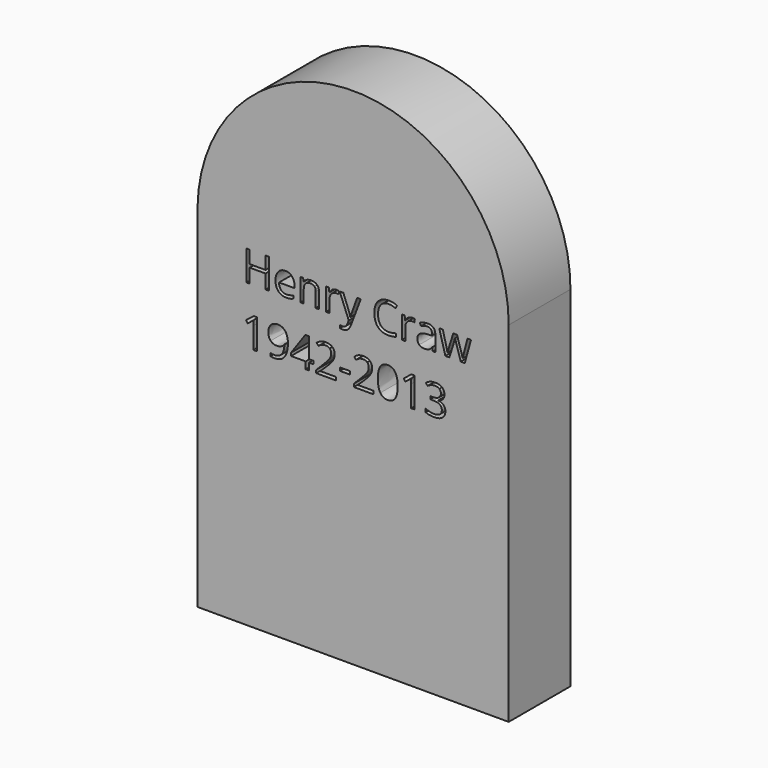
from build123d import *

# Parameters (mm, degrees)
F0_W     = 3.3136069849
F0_H     = 1.0260517065
F1_DEPTH = 25.4


with BuildPart() as f1:
    # F0 (on Front) → F1 (new body)
    with BuildSketch(Plane.XZ):
        with BuildLine():
            ThreePointArc((68.7805563211, 9.0927695855), (17.9996618483, 60.291606621), (-33.6136780679, 9.9320663139))
            Line((-33.6136780679, 9.9320663139), (-33.6136780679, -105.8909147978))
            Line((-33.6136780679, -105.8909147978), (68.7805563211, -105.8909147978))
            Line((68.7805563211, -105.8909147978), (68.7805563211, 9.0927695855))
        make_face()
        with BuildLine():
            Line((-14.1120249478, -15.5934271273), (-14.1120249478, -25.4629644899))
            Line((-14.1120249478, -25.4629644899), (-15.2050400289, -25.4629644899))
            Line((-15.2050400289, -25.4629644899), (-15.2050400289, -18.4296500551))
            add(Edge.make_bspline(
                [(-15.2050400289, -18.4296500551), (-15.2050400289, -17.5504857508), (-15.1510373075, -16.7685263449)],
                knots=[0, 0, 0, 1, 1, 1], degree=2))
            add(Edge.make_bspline(
                [(-15.1510373075, -16.7685263449), (-15.2914443831, -16.9110935294), (-15.4674932549, -17.0655413126)],
                knots=[0, 0, 0, 1, 1, 1], degree=2))
            add(Edge.make_bspline(
                [(-15.4674932549, -17.0655413126), (-15.6435421266, -17.2199890958), (-17.0735341892, -18.3821276603)],
                knots=[0, 0, 0, 1, 1, 1], degree=2))
            Line((-17.0735341892, -18.3821276603), (-17.6675641246, -17.6131289076))
            Line((-17.6675641246, -17.6131289076), (-15.0559925178, -15.5934271273))
            Line((-15.0559925178, -15.5934271273), (-14.1120249478, -15.5934271273))
        make_face(mode=Mode.SUBTRACT)
        Polygon((-10.0877421493, 3.2081603542), (-10.0877421493, -6.6613770083), (-11.2347599518, -6.6613770083), (-11.2347599518, -2.0171429681), (-16.4341419679, -2.0171429681), (-16.4341419679, -6.6613770083), (-17.5811597703, -6.6613770083), (-17.5811597703, 3.2081603542), (-16.4341419679, 3.2081603542), (-16.4341419679, -0.9910912616), (-11.2347599518, -0.9910912616), (-11.2347599518, 3.2081603542), align=None, mode=Mode.SUBTRACT)
        with BuildLine():
            add(Edge.make_bspline(
                [(-4.2759692725, -17.4738018864), (-3.8709488621, -18.462051688), (-3.8709488621, -19.8056393963)],
                knots=[0, 0, 0, 1, 1, 1], degree=2))
            add(Edge.make_bspline(
                [(-3.8709488621, -19.8056393963), (-3.8709488621, -25.5990513478), (-8.353174738, -25.5990513478)],
                knots=[0, 0, 0, 1, 1, 1], degree=2))
            add(Edge.make_bspline(
                [(-8.353174738, -25.5990513478), (-9.1372942527, -25.5990513478), (-9.5952373301, -25.4629644899)],
                knots=[0, 0, 0, 1, 1, 1], degree=2))
            Line((-9.5952373301, -25.4629644899), (-9.5952373301, -24.4973958313))
            add(Edge.make_bspline(
                [(-9.5952373301, -24.4973958313), (-9.0552101162, -24.6723646486), (-8.3682955, -24.6723646486)],
                knots=[0, 0, 0, 1, 1, 1], degree=2))
            add(Edge.make_bspline(
                [(-8.3682955, -24.6723646486), (-6.7482138581, -24.6723646486), (-5.9208921663, -23.6700741395)],
                knots=[0, 0, 0, 1, 1, 1], degree=2))
            add(Edge.make_bspline(
                [(-5.9208921663, -23.6700741395), (-5.0935704745, -22.6677836303), (-5.0201267734, -20.5962392376)],
                knots=[0, 0, 0, 1, 1, 1], degree=2))
            Line((-5.0201267734, -20.5962392376), (-5.1000508011, -20.5962392376))
            add(Edge.make_bspline(
                [(-5.1000508011, -20.5962392376), (-5.4715895243, -21.1557074312), (-6.0861404938, -21.4494822356)],
                knots=[0, 0, 0, 1, 1, 1], degree=2))
            add(Edge.make_bspline(
                [(-6.0861404938, -21.4494822356), (-6.7006914633, -21.74325704), (-7.469690216, -21.74325704)],
                knots=[0, 0, 0, 1, 1, 1], degree=2))
            add(Edge.make_bspline(
                [(-7.469690216, -21.74325704), (-8.7787161826, -21.74325704), (-9.5487949897, -20.9602175798)],
                knots=[0, 0, 0, 1, 1, 1], degree=2))
            add(Edge.make_bspline(
                [(-9.5487949897, -20.9602175798), (-10.3188737969, -20.1771781195), (-10.3188737969, -18.7731073632)],
                knots=[0, 0, 0, 1, 1, 1], degree=2))
            add(Edge.make_bspline(
                [(-10.3188737969, -18.7731073632), (-10.3188737969, -17.2351098578), (-9.4580704178, -16.3440649548)],
                knots=[0, 0, 0, 1, 1, 1], degree=2))
            add(Edge.make_bspline(
                [(-9.4580704178, -16.3440649548), (-8.5972670387, -15.4530200517), (-7.1931962824, -15.4530200517)],
                knots=[0, 0, 0, 1, 1, 1], degree=2))
            add(Edge.make_bspline(
                [(-7.1931962824, -15.4530200517), (-6.1865855556, -15.4530200517), (-5.4337876193, -15.9692860683)],
                knots=[0, 0, 0, 1, 1, 1], degree=2))
            add(Edge.make_bspline(
                [(-5.4337876193, -15.9692860683), (-4.680989683, -16.4855520848), (-4.2759692725, -17.4738018864)],
                knots=[0, 0, 0, 1, 1, 1], degree=2))
        make_face(mode=Mode.SUBTRACT)
        Polygon((4.4973128456, -22.1752788112), (4.4973128456, -23.1948501912), (3.0327590413, -23.1948501912), (3.0327590413, -25.4629644899), (1.95918494, -25.4629644899), (1.95918494, -23.1948501912), (-2.8405769378, -23.1948501912), (-2.8405769378, -22.2163208795), (1.8446991706, -15.5394244059), (3.0327590413, -15.5394244059), (3.0327590413, -22.1752788112), align=None, mode=Mode.SUBTRACT)
        with BuildLine():
            add(Edge.make_bspline(
                [(-3.1451522865, -6.6851382057), (-3.6743789562, -6.7974638662), (-4.4239367292, -6.7974638662)],
                knots=[0, 0, 0, 1, 1, 1], degree=2))
            add(Edge.make_bspline(
                [(-4.4239367292, -6.7974638662), (-6.0634593508, -6.7974638662), (-7.0128271929, -5.7973334659)],
                knots=[0, 0, 0, 1, 1, 1], degree=2))
            add(Edge.make_bspline(
                [(-7.0128271929, -5.7973334659), (-7.9621950351, -4.7972030657), (-7.9621950351, -3.023753695)],
                knots=[0, 0, 0, 1, 1, 1], degree=2))
            add(Edge.make_bspline(
                [(-7.9621950351, -3.023753695), (-7.9621950351, -1.2330234535), (-7.0808706219, -0.1799703862)],
                knots=[0, 0, 0, 1, 1, 1], degree=2))
            add(Edge.make_bspline(
                [(-7.0808706219, -0.1799703862), (-6.1995462087, 0.873082681), (-4.7133913159, 0.873082681)],
                knots=[0, 0, 0, 1, 1, 1], degree=2))
            add(Edge.make_bspline(
                [(-4.7133913159, 0.873082681), (-3.3244413215, 0.873082681), (-2.5144005006, -0.0417234194)],
                knots=[0, 0, 0, 1, 1, 1], degree=2))
            add(Edge.make_bspline(
                [(-2.5144005006, -0.0417234194), (-1.7043596796, -0.9565295199), (-1.7043596796, -2.4556450659)],
                knots=[0, 0, 0, 1, 1, 1], degree=2))
            Line((-1.7043596796, -2.4556450659), (-1.7043596796, -3.1641607706))
            Line((-1.7043596796, -3.1641607706), (-6.8000564706, -3.1641607706))
            add(Edge.make_bspline(
                [(-6.8000564706, -3.1641607706), (-6.7654947289, -4.4667064107), (-6.1412232696, -5.1417404282)],
                knots=[0, 0, 0, 1, 1, 1], degree=2))
            add(Edge.make_bspline(
                [(-6.1412232696, -5.1417404282), (-5.5169518102, -5.8167744456), (-4.3828946609, -5.8167744456)],
                knots=[0, 0, 0, 1, 1, 1], degree=2))
            add(Edge.make_bspline(
                [(-4.3828946609, -5.8167744456), (-3.1883544636, -5.8167744456), (-2.0218956814, -5.3177892999)],
                knots=[0, 0, 0, 1, 1, 1], degree=2))
            Line((-2.0218956814, -5.3177892999), (-2.0218956814, -6.3179197002))
            add(Edge.make_bspline(
                [(-2.0218956814, -6.3179197002), (-2.6159256168, -6.5728125452), (-3.1451522865, -6.6851382057)],
                knots=[0, 0, 0, 1, 1, 1], degree=2))
        make_face(mode=Mode.SUBTRACT)
        with BuildLine():
            Line((6.3917283122, -6.6613770083), (5.270631816, -6.6613770083))
            Line((5.270631816, -6.6613770083), (5.270631816, -1.8745757837))
            add(Edge.make_bspline(
                [(5.270631816, -1.8745757837), (5.270631816, -0.9716502819), (4.859131079, -0.5255878032)],
                knots=[0, 0, 0, 1, 1, 1], degree=2))
            add(Edge.make_bspline(
                [(4.859131079, -0.5255878032), (4.4476303419, -0.0795253244), (3.5684660376, -0.0795253244)],
                knots=[0, 0, 0, 1, 1, 1], degree=2))
            add(Edge.make_bspline(
                [(3.5684660376, -0.0795253244), (2.408487582, -0.0795253244), (1.868460368, -0.707036947)],
                knots=[0, 0, 0, 1, 1, 1], degree=2))
            add(Edge.make_bspline(
                [(1.868460368, -0.707036947), (1.328433154, -1.3345485697), (1.328433154, -2.7796613943)],
                knots=[0, 0, 0, 1, 1, 1], degree=2))
            Line((1.328433154, -2.7796613943), (1.328433154, -6.6613770083))
            Line((1.328433154, -6.6613770083), (0.2073366578, -6.6613770083))
            Line((0.2073366578, -6.6613770083), (0.2073366578, 0.7369958231))
            Line((0.2073366578, 0.7369958231), (1.118902595, 0.7369958231))
            Line((1.118902595, 0.7369958231), (1.3003517389, -0.2760952303))
            Line((1.3003517389, -0.2760952303), (1.3543544603, -0.2760952303))
            add(Edge.make_bspline(
                [(1.3543544603, -0.2760952303), (1.6999718772, 0.2704123102), (2.3210031733, 0.5717474956)],
                knots=[0, 0, 0, 1, 1, 1], degree=2))
            add(Edge.make_bspline(
                [(2.3210031733, 0.5717474956), (2.9420344694, 0.873082681), (3.7045528955, 0.873082681)],
                knots=[0, 0, 0, 1, 1, 1], degree=2))
            add(Edge.make_bspline(
                [(3.7045528955, 0.873082681), (5.0416602773, 0.873082681), (5.7166942948, 0.2282901875)],
                knots=[0, 0, 0, 1, 1, 1], degree=2))
            add(Edge.make_bspline(
                [(5.7166942948, 0.2282901875), (6.3917283122, -0.4165023059), (6.3917283122, -1.8356938242)],
                knots=[0, 0, 0, 1, 1, 1], degree=2))
            Line((6.3917283122, -1.8356938242), (6.3917283122, -6.6613770083))
        make_face(mode=Mode.SUBTRACT)
        with BuildLine():
            Line((11.9367277453, -24.4239521302), (11.9367277453, -25.4629644899))
            Line((11.9367277453, -25.4629644899), (5.4499208511, -25.4629644899))
            Line((5.4499208511, -25.4629644899), (5.4499208511, -24.4973958313))
            Line((5.4499208511, -24.4973958313), (8.0485318047, -21.8858242245))
            add(Edge.make_bspline(
                [(8.0485318047, -21.8858242245), (9.2365916754, -20.6826435918), (9.6146107252, -20.1696177385)],
                knots=[0, 0, 0, 1, 1, 1], degree=2))
            add(Edge.make_bspline(
                [(9.6146107252, -20.1696177385), (9.992629775, -19.6565918853), (10.1816392999, -19.1705673927)],
                knots=[0, 0, 0, 1, 1, 1], degree=2))
            add(Edge.make_bspline(
                [(10.1816392999, -19.1705673927), (10.3706488247, -18.6845429001), (10.3706488247, -18.1250747064)],
                knots=[0, 0, 0, 1, 1, 1], degree=2))
            add(Edge.make_bspline(
                [(10.3706488247, -18.1250747064), (10.3706488247, -17.3344748652), (9.8911046587, -16.87221157)],
                knots=[0, 0, 0, 1, 1, 1], degree=2))
            add(Edge.make_bspline(
                [(9.8911046587, -16.87221157), (9.4115604927, -16.4099482749), (8.5604776035, -16.4099482749)],
                knots=[0, 0, 0, 1, 1, 1], degree=2))
            add(Edge.make_bspline(
                [(8.5604776035, -16.4099482749), (7.9470066885, -16.4099482749), (7.3961789302, -16.6129985073)],
                knots=[0, 0, 0, 1, 1, 1], degree=2))
            add(Edge.make_bspline(
                [(7.3961789302, -16.6129985073), (6.845351172, -16.8160487398), (6.1713972089, -17.3495956272)],
                knots=[0, 0, 0, 1, 1, 1], degree=2))
            Line((6.1713972089, -17.3495956272), (5.5773672736, -16.587077201))
            add(Edge.make_bspline(
                [(5.5773672736, -16.587077201), (6.9403959616, -15.4530200517), (8.5475169504, -15.4530200517)],
                knots=[0, 0, 0, 1, 1, 1], degree=2))
            add(Edge.make_bspline(
                [(8.5475169504, -15.4530200517), (9.9386270536, -15.4530200517), (10.7281468404, -16.1647759197)],
                knots=[0, 0, 0, 1, 1, 1], degree=2))
            add(Edge.make_bspline(
                [(10.7281468404, -16.1647759197), (11.5176666272, -16.8765317877), (11.5176666272, -18.0775523116)],
                knots=[0, 0, 0, 1, 1, 1], degree=2))
            add(Edge.make_bspline(
                [(11.5176666272, -18.0775523116), (11.5176666272, -19.0171996639), (10.9906000664, -19.9352459277)],
                knots=[0, 0, 0, 1, 1, 1], degree=2))
            add(Edge.make_bspline(
                [(10.9906000664, -19.9352459277), (10.4635335055, -20.8532921914), (9.0205807898, -22.2573629477)],
                knots=[0, 0, 0, 1, 1, 1], degree=2))
            Line((9.0205807898, -22.2573629477), (6.8604719339, -24.3699494088))
            Line((6.8604719339, -24.3699494088), (6.8604719339, -24.4239521302))
            Line((6.8604719339, -24.4239521302), (11.9367277453, -24.4239521302))
        make_face(mode=Mode.SUBTRACT)
        with Locations((14.9025572044, -21.7572977476)):
            Rectangle(F0_W, F0_H, mode=Mode.SUBTRACT)
        with BuildLine():
            add(Edge.make_bspline(
                [(10.7918700516, 0.4810229237), (11.3729393339, 0.873082681), (12.0684943855, 0.873082681)],
                knots=[0, 0, 0, 1, 1, 1], degree=2))
            add(Edge.make_bspline(
                [(12.0684943855, 0.873082681), (12.5609992046, 0.873082681), (12.9519789075, 0.7909985445)],
                knots=[0, 0, 0, 1, 1, 1], degree=2))
            Line((12.9519789075, 0.7909985445), (12.7964510699, -0.2480138152))
            add(Edge.make_bspline(
                [(12.7964510699, -0.2480138152), (12.3385079925, -0.1464886989), (11.9864102489, -0.1464886989)],
                knots=[0, 0, 0, 1, 1, 1], degree=2))
            add(Edge.make_bspline(
                [(11.9864102489, -0.1464886989), (11.0878049649, -0.1464886989), (10.4505728524, -0.8755254378)],
                knots=[0, 0, 0, 1, 1, 1], degree=2))
            add(Edge.make_bspline(
                [(10.4505728524, -0.8755254378), (9.8133407399, -1.6045621767), (9.8133407399, -2.6910969312)],
                knots=[0, 0, 0, 1, 1, 1], degree=2))
            Line((9.8133407399, -2.6910969312), (9.8133407399, -6.6613770083))
            Line((9.8133407399, -6.6613770083), (8.6922442437, -6.6613770083))
            Line((8.6922442437, -6.6613770083), (8.6922442437, 0.7369958231))
            Line((8.6922442437, 0.7369958231), (9.616770834, 0.7369958231))
            Line((9.616770834, 0.7369958231), (9.7463773654, -0.6325131915))
            Line((9.7463773654, -0.6325131915), (9.8003800868, -0.6325131915))
            add(Edge.make_bspline(
                [(9.8003800868, -0.6325131915), (10.2108007694, 0.0889631663), (10.7918700516, 0.4810229237)],
                knots=[0, 0, 0, 1, 1, 1], degree=2))
        make_face(mode=Mode.SUBTRACT)
        with BuildLine():
            Line((16.1467799054, -6.7024190765), (13.1615094665, 0.7369958231))
            Line((13.1615094665, 0.7369958231), (14.3646900993, 0.7369958231))
            Line((14.3646900993, 0.7369958231), (15.9847717412, -3.4816967724))
            add(Edge.make_bspline(
                [(15.9847717412, -3.4816967724), (16.5161585197, -4.926809597), (16.6457650511, -5.5683619272)],
                knots=[0, 0, 0, 1, 1, 1], degree=2))
            Line((16.6457650511, -5.5683619272), (16.6997677725, -5.5683619272))
            add(Edge.make_bspline(
                [(16.6997677725, -5.5683619272), (16.7861721267, -5.2227445103), (17.066986278, -4.3889424919)],
                knots=[0, 0, 0, 1, 1, 1], degree=2))
            add(Edge.make_bspline(
                [(17.066986278, -4.3889424919), (17.3478004292, -3.5551404735), (18.9009186966, 0.7369958231)],
                knots=[0, 0, 0, 1, 1, 1], degree=2))
            Line((18.9009186966, 0.7369958231), (20.1019392205, 0.7369958231))
            Line((20.1019392205, 0.7369958231), (16.9222589846, -7.6874287148))
            add(Edge.make_bspline(
                [(16.9222589846, -7.6874287148), (16.4491951452, -8.9359716335), (15.8184433593, -9.4597980311)],
                knots=[0, 0, 0, 1, 1, 1], degree=2))
            add(Edge.make_bspline(
                [(15.8184433593, -9.4597980311), (15.1876915734, -9.9836244286), (14.2696453096, -9.9836244286)],
                knots=[0, 0, 0, 1, 1, 1], degree=2))
            add(Edge.make_bspline(
                [(14.2696453096, -9.9836244286), (13.7555394019, -9.9836244286), (13.2565542562, -9.8669785504)],
                knots=[0, 0, 0, 1, 1, 1], degree=2))
            Line((13.2565542562, -9.8669785504), (13.2565542562, -8.9705333752))
            add(Edge.make_bspline(
                [(13.2565542562, -8.9705333752), (13.6280929794, -9.0504574029), (14.0860360569, -9.0504574029)],
                knots=[0, 0, 0, 1, 1, 1], degree=2))
            add(Edge.make_bspline(
                [(14.0860360569, -9.0504574029), (15.2416942948, -9.0504574029), (15.7341991139, -7.7543920894)],
                knots=[0, 0, 0, 1, 1, 1], degree=2))
            Line((15.7341991139, -7.7543920894), (16.1467799054, -6.7024190765))
        make_face(mode=Mode.SUBTRACT)
        with BuildLine():
            Line((24.2882301832, -24.4239521302), (24.2882301832, -25.4629644899))
            Line((24.2882301832, -25.4629644899), (17.801423289, -25.4629644899))
            Line((17.801423289, -25.4629644899), (17.801423289, -24.4973958313))
            Line((17.801423289, -24.4973958313), (20.4000342426, -21.8858242245))
            add(Edge.make_bspline(
                [(20.4000342426, -21.8858242245), (21.5880941133, -20.6826435918), (21.9661131631, -20.1696177385)],
                knots=[0, 0, 0, 1, 1, 1], degree=2))
            add(Edge.make_bspline(
                [(21.9661131631, -20.1696177385), (22.3441322129, -19.6565918853), (22.5331417378, -19.1705673927)],
                knots=[0, 0, 0, 1, 1, 1], degree=2))
            add(Edge.make_bspline(
                [(22.5331417378, -19.1705673927), (22.7221512627, -18.6845429001), (22.7221512627, -18.1250747064)],
                knots=[0, 0, 0, 1, 1, 1], degree=2))
            add(Edge.make_bspline(
                [(22.7221512627, -18.1250747064), (22.7221512627, -17.3344748652), (22.2426070967, -16.87221157)],
                knots=[0, 0, 0, 1, 1, 1], degree=2))
            add(Edge.make_bspline(
                [(22.2426070967, -16.87221157), (21.7630629307, -16.4099482749), (20.9119800414, -16.4099482749)],
                knots=[0, 0, 0, 1, 1, 1], degree=2))
            add(Edge.make_bspline(
                [(20.9119800414, -16.4099482749), (20.2985091264, -16.4099482749), (19.7476813681, -16.6129985073)],
                knots=[0, 0, 0, 1, 1, 1], degree=2))
            add(Edge.make_bspline(
                [(19.7476813681, -16.6129985073), (19.1968536099, -16.8160487398), (18.5228996468, -17.3495956272)],
                knots=[0, 0, 0, 1, 1, 1], degree=2))
            Line((18.5228996468, -17.3495956272), (17.9288697115, -16.587077201))
            add(Edge.make_bspline(
                [(17.9288697115, -16.587077201), (19.2918983995, -15.4530200517), (20.8990193883, -15.4530200517)],
                knots=[0, 0, 0, 1, 1, 1], degree=2))
            add(Edge.make_bspline(
                [(20.8990193883, -15.4530200517), (22.2901294915, -15.4530200517), (23.0796492783, -16.1647759197)],
                knots=[0, 0, 0, 1, 1, 1], degree=2))
            add(Edge.make_bspline(
                [(23.0796492783, -16.1647759197), (23.8691690651, -16.8765317877), (23.8691690651, -18.0775523116)],
                knots=[0, 0, 0, 1, 1, 1], degree=2))
            add(Edge.make_bspline(
                [(23.8691690651, -18.0775523116), (23.8691690651, -19.0171996639), (23.3421025043, -19.9352459277)],
                knots=[0, 0, 0, 1, 1, 1], degree=2))
            add(Edge.make_bspline(
                [(23.3421025043, -19.9352459277), (22.8150359435, -20.8532921914), (21.3720832277, -22.2573629477)],
                knots=[0, 0, 0, 1, 1, 1], degree=2))
            Line((21.3720832277, -22.2573629477), (19.2119743719, -24.3699494088))
            Line((19.2119743719, -24.3699494088), (19.2119743719, -24.4239521302))
            Line((19.2119743719, -24.4239521302), (24.2882301832, -24.4239521302))
        make_face(mode=Mode.SUBTRACT)
        with BuildLine():
            add(Edge.make_bspline(
                [(31.4122691899, -16.7415249842), (32.2460712082, -18.0451506788), (32.2460712082, -20.514155101)],
                knots=[0, 0, 0, 1, 1, 1], degree=2))
            add(Edge.make_bspline(
                [(32.2460712082, -20.514155101), (32.2460712082, -23.0738840953), (31.4392705506, -24.3364677215)],
                knots=[0, 0, 0, 1, 1, 1], degree=2))
            add(Edge.make_bspline(
                [(31.4392705506, -24.3364677215), (30.6324698929, -25.5990513478), (28.9713461827, -25.5990513478)],
                knots=[0, 0, 0, 1, 1, 1], degree=2))
            add(Edge.make_bspline(
                [(28.9713461827, -25.5990513478), (27.3793459559, -25.5990513478), (26.5487841009, -24.3062261975)],
                knots=[0, 0, 0, 1, 1, 1], degree=2))
            add(Edge.make_bspline(
                [(26.5487841009, -24.3062261975), (25.7182222458, -23.0134010473), (25.7182222458, -20.514155101)],
                knots=[0, 0, 0, 1, 1, 1], degree=2))
            add(Edge.make_bspline(
                [(25.7182222458, -20.514155101), (25.7182222458, -17.937145236), (26.5217827402, -16.6875222628)],
                knots=[0, 0, 0, 1, 1, 1], degree=2))
            add(Edge.make_bspline(
                [(26.5217827402, -16.6875222628), (27.3253432345, -15.4378992897), (28.9713461827, -15.4378992897)],
                knots=[0, 0, 0, 1, 1, 1], degree=2))
            add(Edge.make_bspline(
                [(28.9713461827, -15.4378992897), (30.5784671715, -15.4378992897), (31.4122691899, -16.7415249842)],
                knots=[0, 0, 0, 1, 1, 1], degree=2))
        make_face(mode=Mode.SUBTRACT)
        with BuildLine():
            Line((37.7586690084, -15.5934271273), (37.7586690084, -25.4629644899))
            Line((37.7586690084, -25.4629644899), (36.6656539274, -25.4629644899))
            Line((36.6656539274, -25.4629644899), (36.6656539274, -18.4296500551))
            add(Edge.make_bspline(
                [(36.6656539274, -18.4296500551), (36.6656539274, -17.5504857508), (36.7196566488, -16.7685263449)],
                knots=[0, 0, 0, 1, 1, 1], degree=2))
            add(Edge.make_bspline(
                [(36.7196566488, -16.7685263449), (36.5792495731, -16.9110935294), (36.4032007014, -17.0655413126)],
                knots=[0, 0, 0, 1, 1, 1], degree=2))
            add(Edge.make_bspline(
                [(36.4032007014, -17.0655413126), (36.2271518296, -17.2199890958), (34.797159767, -18.3821276603)],
                knots=[0, 0, 0, 1, 1, 1], degree=2))
            Line((34.797159767, -18.3821276603), (34.2031298317, -17.6131289076))
            Line((34.2031298317, -17.6131289076), (36.8147014384, -15.5934271273))
            Line((36.8147014384, -15.5934271273), (37.7586690084, -15.5934271273))
        make_face(mode=Mode.SUBTRACT)
        with BuildLine():
            add(Edge.make_bspline(
                [(35.7173661396, 0.4810229237), (36.2984354219, 0.873082681), (36.9939904735, 0.873082681)],
                knots=[0, 0, 0, 1, 1, 1], degree=2))
            add(Edge.make_bspline(
                [(36.9939904735, 0.873082681), (37.4864952926, 0.873082681), (37.8774749955, 0.7909985445)],
                knots=[0, 0, 0, 1, 1, 1], degree=2))
            Line((37.8774749955, 0.7909985445), (37.7219471579, -0.2480138152))
            add(Edge.make_bspline(
                [(37.7219471579, -0.2480138152), (37.2640040804, -0.1464886989), (36.9119063369, -0.1464886989)],
                knots=[0, 0, 0, 1, 1, 1], degree=2))
            add(Edge.make_bspline(
                [(36.9119063369, -0.1464886989), (36.0133010529, -0.1464886989), (35.3760689404, -0.8755254378)],
                knots=[0, 0, 0, 1, 1, 1], degree=2))
            add(Edge.make_bspline(
                [(35.3760689404, -0.8755254378), (34.7388368279, -1.6045621767), (34.7388368279, -2.6910969312)],
                knots=[0, 0, 0, 1, 1, 1], degree=2))
            Line((34.7388368279, -2.6910969312), (34.7388368279, -6.6613770083))
            Line((34.7388368279, -6.6613770083), (33.6177403317, -6.6613770083))
            Line((33.6177403317, -6.6613770083), (33.6177403317, 0.7369958231))
            Line((33.6177403317, 0.7369958231), (34.542266922, 0.7369958231))
            Line((34.542266922, 0.7369958231), (34.6718734534, -0.6325131915))
            Line((34.6718734534, -0.6325131915), (34.7258761748, -0.6325131915))
            add(Edge.make_bspline(
                [(34.7258761748, -0.6325131915), (35.1362968574, 0.0889631663), (35.7173661396, 0.4810229237)],
                knots=[0, 0, 0, 1, 1, 1], degree=2))
        make_face(mode=Mode.SUBTRACT)
        with BuildLine():
            Line((44.6429359321, -6.6613770083), (43.8112940226, -6.6613770083))
            Line((43.8112940226, -6.6613770083), (43.5888028105, -5.6072438866))
            Line((43.5888028105, -5.6072438866), (43.5348000891, -5.6072438866))
            add(Edge.make_bspline(
                [(43.5348000891, -5.6072438866), (42.981812222, -6.3027989382), (42.4320645181, -6.5501314022)],
                knots=[0, 0, 0, 1, 1, 1], degree=2))
            add(Edge.make_bspline(
                [(42.4320645181, -6.5501314022), (41.8823168143, -6.7974638662), (41.0571552314, -6.7974638662)],
                knots=[0, 0, 0, 1, 1, 1], degree=2))
            add(Edge.make_bspline(
                [(41.0571552314, -6.7974638662), (39.9576598237, -6.7974638662), (39.3333883644, -6.2293552371)],
                knots=[0, 0, 0, 1, 1, 1], degree=2))
            add(Edge.make_bspline(
                [(39.3333883644, -6.2293552371), (38.709116905, -5.661246608), (38.709116905, -4.6157539218)],
                knots=[0, 0, 0, 1, 1, 1], degree=2))
            add(Edge.make_bspline(
                [(38.709116905, -4.6157539218), (38.709116905, -2.3757210382), (42.2927374969, -2.2677155954)],
                knots=[0, 0, 0, 1, 1, 1], degree=2))
            Line((42.2927374969, -2.2677155954), (43.5477607422, -2.2266735272))
            Line((43.5477607422, -2.2266735272), (43.5477607422, -1.7665703409))
            add(Edge.make_bspline(
                [(43.5477607422, -1.7665703409), (43.5477607422, -0.8960464719), (43.1740619101, -0.4813055716)],
                knots=[0, 0, 0, 1, 1, 1], degree=2))
            add(Edge.make_bspline(
                [(43.1740619101, -0.4813055716), (42.8003630781, -0.0665646713), (41.9752014951, -0.0665646713)],
                knots=[0, 0, 0, 1, 1, 1], degree=2))
            add(Edge.make_bspline(
                [(41.9752014951, -0.0665646713), (41.0506749048, -0.0665646713), (39.8842161226, -0.6325131915)],
                knots=[0, 0, 0, 1, 1, 1], degree=2))
            Line((39.8842161226, -0.6325131915), (39.5385987057, 0.2250500243))
            add(Edge.make_bspline(
                [(39.5385987057, 0.2250500243), (40.0851062462, 0.5209849375), (40.7363790663, 0.6894734283)],
                knots=[0, 0, 0, 1, 1, 1], degree=2))
            add(Edge.make_bspline(
                [(40.7363790663, 0.6894734283), (41.3876518863, 0.857961919), (42.0443249785, 0.857961919)],
                knots=[0, 0, 0, 1, 1, 1], degree=2))
            add(Edge.make_bspline(
                [(42.0443249785, 0.857961919), (43.3663115983, 0.857961919), (44.0046237652, 0.2714923647)],
                knots=[0, 0, 0, 1, 1, 1], degree=2))
            add(Edge.make_bspline(
                [(44.0046237652, 0.2714923647), (44.6429359321, -0.3149771897), (44.6429359321, -1.6110425032)],
                knots=[0, 0, 0, 1, 1, 1], degree=2))
            Line((44.6429359321, -1.6110425032), (44.6429359321, -6.6613770083))
        make_face(mode=Mode.SUBTRACT)
        with BuildLine():
            add(Edge.make_bspline(
                [(31.5310751769, 1.7976092713), (30.4099786807, 2.3225157233), (29.2888821845, 2.3225157233)],
                knots=[0, 0, 0, 1, 1, 1], degree=2))
            add(Edge.make_bspline(
                [(29.2888821845, 2.3225157233), (27.6623202161, 2.3225157233), (26.7205127549, 1.2392211321)],
                knots=[0, 0, 0, 1, 1, 1], degree=2))
            add(Edge.make_bspline(
                [(26.7205127549, 1.2392211321), (25.7787052937, 0.1559265409), (25.7787052937, -1.7276883815)],
                knots=[0, 0, 0, 1, 1, 1], degree=2))
            add(Edge.make_bspline(
                [(25.7787052937, -1.7276883815), (25.7787052937, -3.6631459163), (26.6870310676, -4.7205192013)],
                knots=[0, 0, 0, 1, 1, 1], degree=2))
            add(Edge.make_bspline(
                [(26.6870310676, -4.7205192013), (27.5953568415, -5.7778924862), (29.2759215314, -5.7778924862)],
                knots=[0, 0, 0, 1, 1, 1], degree=2))
            add(Edge.make_bspline(
                [(29.2759215314, -5.7778924862), (30.3084535645, -5.7778924862), (31.6326002932, -5.406353763)],
                knots=[0, 0, 0, 1, 1, 1], degree=2))
            Line((31.6326002932, -5.406353763), (31.6326002932, -6.410804381))
            add(Edge.make_bspline(
                [(31.6326002932, -6.410804381), (30.6065485866, -6.7974638662), (29.1009527141, -6.7974638662)],
                knots=[0, 0, 0, 1, 1, 1], degree=2))
            add(Edge.make_bspline(
                [(29.1009527141, -6.7974638662), (26.9214028785, -6.7974638662), (25.736583171, -5.4733171375)],
                knots=[0, 0, 0, 1, 1, 1], degree=2))
            add(Edge.make_bspline(
                [(25.736583171, -5.4733171375), (24.5517634636, -4.1491704089), (24.5517634636, -1.7125676195)],
                knots=[0, 0, 0, 1, 1, 1], degree=2))
            add(Edge.make_bspline(
                [(24.5517634636, -1.7125676195), (24.5517634636, -0.1875307672), (25.1220322015, 0.9594870353)],
                knots=[0, 0, 0, 1, 1, 1], degree=2))
            add(Edge.make_bspline(
                [(25.1220322015, 0.9594870353), (25.6923009395, 2.1065048377), (26.7691152042, 2.7275361338)],
                knots=[0, 0, 0, 1, 1, 1], degree=2))
            add(Edge.make_bspline(
                [(26.7691152042, 2.7275361338), (27.8459294688, 3.3485674299), (29.3040029465, 3.3485674299)],
                knots=[0, 0, 0, 1, 1, 1], degree=2))
            add(Edge.make_bspline(
                [(29.3040029465, 3.3485674299), (30.8549611051, 3.3485674299), (32.0170996695, 2.7826189096)],
                knots=[0, 0, 0, 1, 1, 1], degree=2))
            Line((32.0170996695, 2.7826189096), (31.5310751769, 1.7976092713))
        make_face(mode=Mode.SUBTRACT)
        with BuildLine():
            add(Edge.make_bspline(
                [(46.8311262031, -16.1107731983), (47.628206371, -16.7685263449), (47.628206371, -17.9155441474)],
                knots=[0, 0, 0, 1, 1, 1], degree=2))
            add(Edge.make_bspline(
                [(47.628206371, -17.9155441474), (47.628206371, -18.8616718263), (47.0978996468, -19.4621820882)],
                knots=[0, 0, 0, 1, 1, 1], degree=2))
            add(Edge.make_bspline(
                [(47.0978996468, -19.4621820882), (46.5675929227, -20.0626923502), (45.5955439376, -20.2657425826)],
                knots=[0, 0, 0, 1, 1, 1], degree=2))
            Line((45.5955439376, -20.2657425826), (45.5955439376, -20.319745304))
            add(Edge.make_bspline(
                [(45.5955439376, -20.319745304), (46.7836038083, -20.4666327062), (47.3571127095, -21.0747033491)],
                knots=[0, 0, 0, 1, 1, 1], degree=2))
            add(Edge.make_bspline(
                [(47.3571127095, -21.0747033491), (47.9306216108, -21.6827739921), (47.9306216108, -22.6677836303)],
                knots=[0, 0, 0, 1, 1, 1], degree=2))
            add(Edge.make_bspline(
                [(47.9306216108, -22.6677836303), (47.9306216108, -24.0783347132), (46.9520922991, -24.8386930305)],
                knots=[0, 0, 0, 1, 1, 1], degree=2))
            add(Edge.make_bspline(
                [(46.9520922991, -24.8386930305), (45.9735629874, -25.5990513478), (44.1720322015, -25.5990513478)],
                knots=[0, 0, 0, 1, 1, 1], degree=2))
            add(Edge.make_bspline(
                [(44.1720322015, -25.5990513478), (43.3879126869, -25.5990513478), (42.7366398668, -25.4802453607)],
                knots=[0, 0, 0, 1, 1, 1], degree=2))
            add(Edge.make_bspline(
                [(42.7366398668, -25.4802453607), (42.0853670468, -25.3614393736), (41.4718961317, -25.0655044604)],
                knots=[0, 0, 0, 1, 1, 1], degree=2))
            Line((41.4718961317, -25.0655044604), (41.4718961317, -23.9984106856))
            add(Edge.make_bspline(
                [(41.4718961317, -23.9984106856), (42.1134484619, -24.3159466874), (42.8392450375, -24.4811950149)],
                knots=[0, 0, 0, 1, 1, 1], degree=2))
            add(Edge.make_bspline(
                [(42.8392450375, -24.4811950149), (43.565041613, -24.6464433423), (44.2130742698, -24.6464433423)],
                knots=[0, 0, 0, 1, 1, 1], degree=2))
            add(Edge.make_bspline(
                [(44.2130742698, -24.6464433423), (46.7706431552, -24.6464433423), (46.7706431552, -22.6418623241)],
                knots=[0, 0, 0, 1, 1, 1], degree=2))
            add(Edge.make_bspline(
                [(46.7706431552, -22.6418623241), (46.7706431552, -20.844651756), (43.9495409894, -20.844651756)],
                knots=[0, 0, 0, 1, 1, 1], degree=2))
            Line((43.9495409894, -20.844651756), (42.9774920042, -20.844651756))
            Line((42.9774920042, -20.844651756), (42.9774920042, -19.8812432063))
            Line((42.9774920042, -19.8812432063), (43.9625016425, -19.8812432063))
            add(Edge.make_bspline(
                [(43.9625016425, -19.8812432063), (45.1159997716, -19.8812432063), (45.791033789, -19.3714575163)],
                knots=[0, 0, 0, 1, 1, 1], degree=2))
            add(Edge.make_bspline(
                [(45.791033789, -19.3714575163), (46.4660678065, -18.8616718263), (46.4660678065, -17.9565862157)],
                knots=[0, 0, 0, 1, 1, 1], degree=2))
            add(Edge.make_bspline(
                [(46.4660678065, -17.9565862157), (46.4660678065, -17.2351098578), (45.9703228241, -16.8225290663)],
                knots=[0, 0, 0, 1, 1, 1], degree=2))
            add(Edge.make_bspline(
                [(45.9703228241, -16.8225290663), (45.4745778416, -16.4099482749), (44.6234949524, -16.4099482749)],
                knots=[0, 0, 0, 1, 1, 1], degree=2))
            add(Edge.make_bspline(
                [(44.6234949524, -16.4099482749), (43.9754622957, -16.4099482749), (43.4019533944, -16.5859971466)],
                knots=[0, 0, 0, 1, 1, 1], degree=2))
            add(Edge.make_bspline(
                [(43.4019533944, -16.5859971466), (42.8284444932, -16.7620460184), (42.0918473733, -17.2351098578)],
                knots=[0, 0, 0, 1, 1, 1], degree=2))
            Line((42.0918473733, -17.2351098578), (41.5258988531, -16.4790717583))
            add(Edge.make_bspline(
                [(41.5258988531, -16.4790717583), (42.1328894416, -15.9995275922), (42.9256493917, -15.726273822)],
                knots=[0, 0, 0, 1, 1, 1], degree=2))
            add(Edge.make_bspline(
                [(42.9256493917, -15.726273822), (43.7184093418, -15.4530200517), (44.5975736462, -15.4530200517)],
                knots=[0, 0, 0, 1, 1, 1], degree=2))
            add(Edge.make_bspline(
                [(44.5975736462, -15.4530200517), (46.0340460353, -15.4530200517), (46.8311262031, -16.1107731983)],
                knots=[0, 0, 0, 1, 1, 1], degree=2))
        make_face(mode=Mode.SUBTRACT)
        with BuildLine():
            Line((54.3223837153, -6.6613770083), (52.9917566601, -6.6613770083))
            Line((52.9917566601, -6.6613770083), (51.6352082986, -2.3217183168))
            add(Edge.make_bspline(
                [(51.6352082986, -2.3217183168), (51.5056017673, -1.9220981785), (51.1556641326, -0.5115470956)],
                knots=[0, 0, 0, 1, 1, 1], degree=2))
            Line((51.1556641326, -0.5115470956), (51.1016614112, -0.5115470956))
            add(Edge.make_bspline(
                [(51.1016614112, -0.5115470956), (50.8316478042, -1.6931266398), (50.6285975718, -2.33467897)],
                knots=[0, 0, 0, 1, 1, 1], degree=2))
            Line((50.6285975718, -2.33467897), (49.231007142, -6.6613770083))
            Line((49.231007142, -6.6613770083), (47.9349418285, -6.6613770083))
            Line((47.9349418285, -6.6613770083), (45.9174001571, 0.7369958231))
            Line((45.9174001571, 0.7369958231), (47.0924993747, 0.7369958231))
            add(Edge.make_bspline(
                [(47.0924993747, 0.7369958231), (47.807495406, -2.0517047098), (48.1822742925, -3.5097781876)],
                knots=[0, 0, 0, 1, 1, 1], degree=2))
            add(Edge.make_bspline(
                [(48.1822742925, -3.5097781876), (48.557053179, -4.9678516653), (48.6110559004, -5.4733171375)],
                knots=[0, 0, 0, 1, 1, 1], degree=2))
            Line((48.6110559004, -5.4733171375), (48.6650586218, -5.4733171375))
            add(Edge.make_bspline(
                [(48.6650586218, -5.4733171375), (48.7385023229, -5.0888177612), (48.9037506504, -4.477506955)],
                knots=[0, 0, 0, 1, 1, 1], degree=2))
            add(Edge.make_bspline(
                [(48.9037506504, -4.477506955), (49.0689989778, -3.8661961488), (49.1921251826, -3.5097781876)],
                knots=[0, 0, 0, 1, 1, 1], degree=2))
            Line((49.1921251826, -3.5097781876), (50.5486735441, 0.7369958231))
            Line((50.5486735441, 0.7369958231), (51.7626547211, 0.7369958231))
            Line((51.7626547211, 0.7369958231), (53.0868014498, -3.5097781876))
            add(Edge.make_bspline(
                [(53.0868014498, -3.5097781876), (53.4648204995, -4.6697566432), (53.5987472486, -5.4603564844)],
                knots=[0, 0, 0, 1, 1, 1], degree=2))
            Line((53.5987472486, -5.4603564844), (53.65274997, -5.4603564844))
            add(Edge.make_bspline(
                [(53.65274997, -5.4603564844), (53.6808313851, -5.2162641837), (53.7985573178, -4.709718657)],
                knots=[0, 0, 0, 1, 1, 1], degree=2))
            add(Edge.make_bspline(
                [(53.7985573178, -4.709718657), (53.9162832504, -4.2031731303), (55.2058682374, 0.7369958231)],
                knots=[0, 0, 0, 1, 1, 1], degree=2))
            Line((55.2058682374, 0.7369958231), (56.365846693, 0.7369958231))
            Line((56.365846693, 0.7369958231), (54.3223837153, -6.6613770083))
        make_face(mode=Mode.SUBTRACT)
    extrude(amount=-F1_DEPTH)


solid = f1.part
